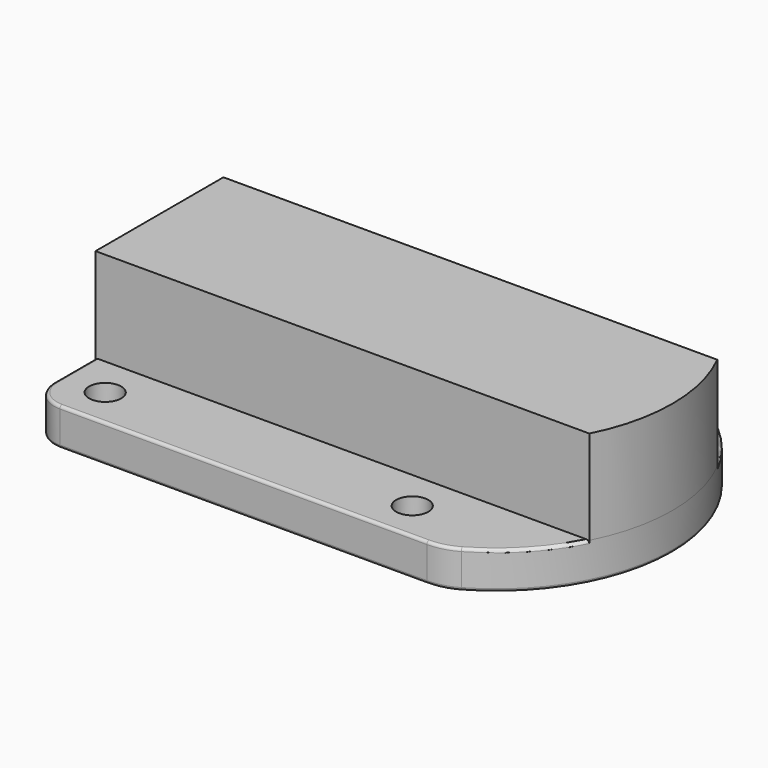
from build123d import *

# Parameters (mm, degrees)
F0_R         = 2.8
F1_DEPTH     = 6.5
F3_DEPTH     = 16.35
F4_T1_DEPTH  = 63.8184719387
F4_T3_DEPTH  = 45.8
F4_T5_DEPTH  = 9
F4_T7_DEPTH  = 9
F4_T10_ANGLE = 90
F4_T12_ANGLE = 120.4504110916
F4_T14_ANGLE = 90
F4_T16_ANGLE = 90
F4_T18_ANGLE = 29.7747944542
F4_T20_ANGLE = 29.7747944542
F4_T22_ANGLE = 29.7747944542
F4_T26_ANGLE = 35.5690080159
F4_T29_ANGLE = 90
F4_T33_ANGLE = 35.5690080159
F4_T36_ANGLE = 29.7747944542
F5_SIZE      = 1.56


# Not quite as in the source:
# - a fillet or chamfer that OpenCascade refuses, or shapes differently, is made with other operations: its cross-section is extruded or revolved along the edge and cut away or added


with BuildPart() as f1:
    # F0 (on Top) → F1 (new body)
    with BuildSketch(Plane.XY):
        with BuildLine():
            Line((-38.8770699501, 16.9000072956), (-38.8770699501, -28.8999927044))
            ThreePointArc((-38.8770699501, -28.8999927044), (-37.412603856, -32.4355266103), (-33.8770699501, -33.8999927044))
            Line((-33.8770699501, -33.8999927044), (29.9414019886, -33.8999927044))
            ThreePointArc((29.9414019886, -33.8999927044), (32.5106042183, -33.5643188528), (34.9073236464, -32.579832685))
            ThreePointArc((34.9073236464, -32.579832685), (50.3229300499, -5.9999927044), (34.9073236464, 20.5798472762))
            ThreePointArc((34.9073236464, 20.5798472762), (32.5106042183, 21.564333444), (29.9414019886, 21.9000072956))
            Line((29.9414019886, 21.9000072956), (-33.8770699501, 21.9000072956))
            ThreePointArc((-33.8770699501, 21.9000072956), (-37.412603856, 20.4355412015), (-38.8770699501, 16.9000072956))
        make_face()
        with Locations((-31.5170697868, -26.9999932498)):
            Circle(F0_R, mode=Mode.SUBTRACT)
        with Locations((21.8729300499, -26.9999927044)):
            Circle(F0_R, mode=Mode.SUBTRACT)
        with Locations((-31.5170697868, 15.0000071153)):
            Circle(F0_R, mode=Mode.SUBTRACT)
        with Locations((21.8729300499, 15.0000072956)):
            Circle(F0_R, mode=Mode.SUBTRACT)
    extrude(amount=F1_DEPTH)

    # F2 (on face) → F3 (join)
    with BuildSketch(Plane.XY.offset(6.5)):
        with BuildLine():
            Line((-38.8770699501, 7.9000072956), (-38.8770699501, -5.9999927044))
            Line((-38.8770699501, -5.9999927044), (-38.8770699501, -19.8999927044))
            Line((-38.8770699501, -19.8999927044), (46.9864613892, -19.8999927044))
            ThreePointArc((46.9864613892, -19.8999927044), (50.3229300499, -5.9999927044), (46.9864613892, 7.9000072956))
            Line((46.9864613892, 7.9000072956), (-38.8770699501, 7.9000072956))
        make_face()
    extrude(amount=F3_DEPTH)

    # F4: fillet of radius 0.5 on 18 edges, made by hand

    # F4_s2 → F4_t1 (cut)
    with BuildSketch(Plane.YZ.offset(-33.8770699501)):
        with BuildLine():
            ThreePointArc((21.9000072956, 0.5), (21.7535606862, 0.1464466094), (21.4000072956, 0))
            Line((21.4000072956, 0), (21.9000072956, 0))
            Line((21.9000072956, 0), (21.9000072956, 0.5))
        make_face()
        with BuildLine():
            ThreePointArc((21.9000072956, 6), (21.7535606862, 6.3535533906), (21.4000072956, 6.5))
            Line((21.4000072956, 6.5), (21.9000072956, 6.5))
            Line((21.9000072956, 6.5), (21.9000072956, 6))
        make_face()
        with BuildLine():
            ThreePointArc((-33.3999927044, 6.5), (-33.753546095, 6.3535533906), (-33.8999927044, 6))
            Line((-33.8999927044, 6), (-33.8999927044, 6.5))
            Line((-33.8999927044, 6.5), (-33.3999927044, 6.5))
        make_face()
        with BuildLine():
            ThreePointArc((-33.3999927044, 0), (-33.753546095, 0.1464466094), (-33.8999927044, 0.5))
            Line((-33.8999927044, 0.5), (-33.8999927044, 0))
            Line((-33.8999927044, 0), (-33.3999927044, 0))
        make_face()
    extrude(amount=F4_T1_DEPTH, mode=Mode.SUBTRACT)

    # F4_s4 → F4_t3 (cut)
    with BuildSketch(Plane.XZ.offset(-16.9000072956)):
        with BuildLine():
            ThreePointArc((-38.8770699501, 0.5), (-38.7306233407, 0.1464466094), (-38.3770699501, 0))
            Line((-38.3770699501, 0), (-38.8770699501, 0))
            Line((-38.8770699501, 0), (-38.8770699501, 0.5))
        make_face()
    extrude(amount=F4_T3_DEPTH, mode=Mode.SUBTRACT)

    # F4_s6 → F4_t5 (cut)
    with BuildSketch(Plane.XZ.offset(-16.9000072956)):
        with BuildLine():
            ThreePointArc((-38.8770699501, 6), (-38.7306233407, 6.3535533906), (-38.3770699501, 6.5))
            Line((-38.3770699501, 6.5), (-38.8770699501, 6.5))
            Line((-38.8770699501, 6.5), (-38.8770699501, 6))
        make_face()
    extrude(amount=F4_T5_DEPTH, mode=Mode.SUBTRACT)

    # F4_s8 → F4_t7 (cut)
    with BuildSketch(Plane.XZ.offset(19.8999927044)):
        with BuildLine():
            ThreePointArc((-38.8770699501, 6), (-38.7306233407, 6.3535533906), (-38.3770699501, 6.5))
            Line((-38.3770699501, 6.5), (-38.8770699501, 6.5))
            Line((-38.8770699501, 6.5), (-38.8770699501, 6))
        make_face()
    extrude(amount=F4_T7_DEPTH, mode=Mode.SUBTRACT)

    # F4_s9 → F4_t10 (revolve, cut)
    with BuildSketch(Plane.YZ.offset(-33.8770699501)):
        with BuildLine():
            ThreePointArc((21.9000072956, 0.5), (21.7535606862, 0.1464466094), (21.4000072956, 0))
            Line((21.4000072956, 0), (21.9000072956, 0))
            Line((21.9000072956, 0), (21.9000072956, 0.5))
        make_face()
    revolve(axis=Axis((-33.8770699501, 16.9000072956, 0), (0, 0, 1)), revolution_arc=F4_T10_ANGLE, mode=Mode.SUBTRACT)

    # F4_s11 → F4_t12 (revolve, cut)
    with BuildSketch(Plane(origin=(12.2560283734, 7.0119353437, 0), x_dir=(0, 0, 1), z_dir=(-0.8679839981, -0.4965921658, 0))):
        with BuildLine():
            ThreePointArc((0, -45.1134768811), (0.1464466094, -45.4670302717), (0.5, -45.6134768811))
            Line((0.5, -45.6134768811), (0, -45.6134768811))
            Line((0, -45.6134768811), (0, -45.1134768811))
        make_face()
    revolve(axis=Axis((19.7004300499, -5.9999927044, 0), (0, 0, 1)), revolution_arc=F4_T12_ANGLE, mode=Mode.SUBTRACT)

    # F4_s13 → F4_t14 (revolve, cut)
    with BuildSketch(Plane.YZ.offset(-33.8770699501)):
        with BuildLine():
            ThreePointArc((21.9000072956, 6), (21.7535606862, 6.3535533906), (21.4000072956, 6.5))
            Line((21.4000072956, 6.5), (21.9000072956, 6.5))
            Line((21.9000072956, 6.5), (21.9000072956, 6))
        make_face()
    revolve(axis=Axis((-33.8770699501, 16.9000072956, 6.5), (0, 0, 1)), revolution_arc=F4_T14_ANGLE, mode=Mode.SUBTRACT)

    # F4_s15 → F4_t16 (revolve, cut)
    with BuildSketch(Plane.XZ.offset(28.8999927044)):
        with BuildLine():
            ThreePointArc((-38.3770699501, 0), (-38.7306233407, 0.1464466094), (-38.8770699501, 0.5))
            Line((-38.8770699501, 0.5), (-38.8770699501, 0))
            Line((-38.8770699501, 0), (-38.3770699501, 0))
        make_face()
    revolve(axis=Axis((-33.8770699501, -28.8999927044, 0), (0, 0, 1)), revolution_arc=F4_T16_ANGLE, mode=Mode.SUBTRACT)

    # F4_s17 → F4_t18 (revolve, cut)
    with BuildSketch(Plane.YZ.offset(29.9414019886)):
        with BuildLine():
            ThreePointArc((-33.3999927044, 0), (-33.753546095, 0.1464466094), (-33.8999927044, 0.5))
            Line((-33.8999927044, 0.5), (-33.8999927044, 0))
            Line((-33.8999927044, 0), (-33.3999927044, 0))
        make_face()
    revolve(axis=Axis((29.9414019886, -23.8999927044, 0), (0, 0, 1)), revolution_arc=F4_T18_ANGLE, mode=Mode.SUBTRACT)

    # F4_s19 → F4_t20 (revolve, cut)
    with BuildSketch(Plane(origin=(17.4284307256, -9.9711770948, 0), x_dir=(0, 0, 1), z_dir=(0.8679839981, -0.4965921658, 0))):
        with BuildLine():
            ThreePointArc((0, -34.6976815693), (0.1464466094, -35.0512349599), (0.5, -35.1976815693))
            Line((0.5, -35.1976815693), (0, -35.1976815693))
            Line((0, -35.1976815693), (0, -34.6976815693))
        make_face()
    revolve(axis=Axis((29.9414019886, 11.9000072956, 0), (0, 0, 1)), revolution_arc=F4_T20_ANGLE, mode=Mode.SUBTRACT)

    # F4_s21 → F4_t22 (revolve, cut)
    with BuildSketch(Plane(origin=(17.4284307256, -9.9711770948, 0), x_dir=(0, 0, 1), z_dir=(0.8679839981, -0.4965921658, 0))):
        with BuildLine():
            ThreePointArc((6.5, -34.6976815693), (6.3535533906, -35.0512349599), (6, -35.1976815693))
            Line((6, -35.1976815693), (6.5, -35.1976815693))
            Line((6.5, -35.1976815693), (6.5, -34.6976815693))
        make_face()
    revolve(axis=Axis((29.9414019886, 11.9000072956, 6.5), (0, 0, 1)), revolution_arc=F4_T22_ANGLE, mode=Mode.SUBTRACT)


with BuildPart() as f4_tool24:
    # F4_s25 → F4_t26 (revolve)
    with BuildSketch(Plane(origin=(5.7033446243, -12.4249727464, 0), x_dir=(0, 0, 1), z_dir=(0.4171723997, -0.9088273703, 0))):
        with BuildLine():
            ThreePointArc((6.5, -45.5237586807), (6.3535533906, -45.8773120713), (6, -46.0237586807))
            Line((6, -46.0237586807), (6.5, -46.0237586807))
            Line((6.5, -46.0237586807), (6.5, -45.5237586807))
        make_face()
    revolve(axis=Axis((19.7004300499, -5.9999927044, 6.5), (0, 0, 1)), revolution_arc=F4_T26_ANGLE)

    split(bisect_by=Plane.XZ.offset(-7.9000072956), keep=Keep.BOTTOM)


with BuildPart() as f1_1:
    add(f1.part)

    # F4_t23: cut F4_tool24
    add(f4_tool24.part, mode=Mode.SUBTRACT)

    # F4_s28 → F4_t29 (revolve, cut)
    with BuildSketch(Plane.XZ.offset(28.8999927044)):
        with BuildLine():
            ThreePointArc((-38.8770699501, 6), (-38.7306233407, 6.3535533906), (-38.3770699501, 6.5))
            Line((-38.3770699501, 6.5), (-38.8770699501, 6.5))
            Line((-38.8770699501, 6.5), (-38.8770699501, 6))
        make_face()
    revolve(axis=Axis((-33.8770699501, -28.8999927044, 6.5), (0, 0, 1)), revolution_arc=F4_T29_ANGLE, mode=Mode.SUBTRACT)


with BuildPart() as f4_tool31:
    # F4_s32 → F4_t33 (revolve)
    with BuildSketch(Plane(origin=(12.2560283734, 7.0119353437, 0), x_dir=(0, 0, 1), z_dir=(-0.8679839981, -0.4965921658, 0))):
        with BuildLine():
            ThreePointArc((6.5, -45.1134768811), (6.3535533906, -45.4670302717), (6, -45.6134768811))
            Line((6, -45.6134768811), (6.5, -45.6134768811))
            Line((6.5, -45.6134768811), (6.5, -45.1134768811))
        make_face()
    revolve(axis=Axis((19.7004300499, -5.9999927044, 6.5), (0, 0, 1)), revolution_arc=F4_T33_ANGLE)

    split(bisect_by=Plane.XZ.offset(19.8999927044), keep=Keep.TOP)


with BuildPart() as f1_2:
    add(f1_1.part)

    # F4_t30: cut F4_tool31
    add(f4_tool31.part, mode=Mode.SUBTRACT)

    # F4_s35 → F4_t36 (revolve, cut)
    with BuildSketch(Plane.YZ.offset(29.9414019886)):
        with BuildLine():
            ThreePointArc((-33.3999927044, 6.5), (-33.753546095, 6.3535533906), (-33.8999927044, 6))
            Line((-33.8999927044, 6), (-33.8999927044, 6.5))
            Line((-33.8999927044, 6.5), (-33.3999927044, 6.5))
        make_face()
    revolve(axis=Axis((29.9414019886, -23.8999927044, 6.5), (0, 0, 1)), revolution_arc=F4_T36_ANGLE, mode=Mode.SUBTRACT)

    # F5
    f5_edges = [f1_2.edges().sort_by_distance(p)[0] for p in [
        (-34.31707, 15.000007, 0),
        (-34.31707, -26.999993, 0),
        (19.07293, -26.999993, 0),
        (19.07293, 15.000007, 0),
    ]]
    chamfer(f5_edges, length=F5_SIZE)


solid = f1_2.part
